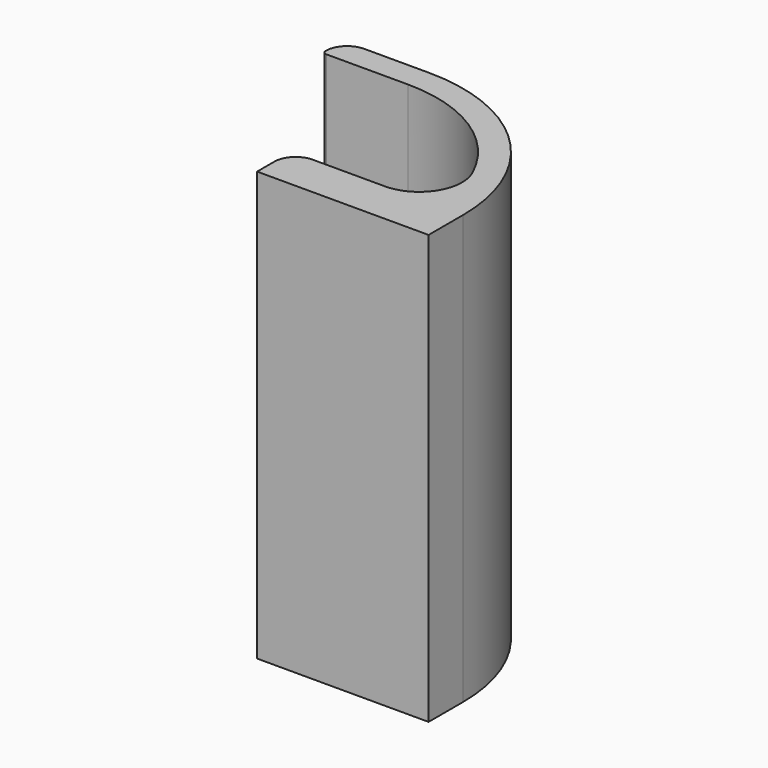
from build123d import *

# Parameters (mm, degrees)
F1_DEPTH = 50
F2_R     = 5
F3_R     = 2.5
F4_R     = 0.49999


# Not quite as in the source:
# - a fillet or chamfer is up to 0.001 mm smaller than in the source, because OpenCascade refuses the exact size


with BuildPart() as f1:
    # F0 (on Top) → F1 (new body)
    with BuildSketch(Plane.XY):
        with BuildLine():
            Line((7, 2.5), (10, 2.5))
            ThreePointArc((10, 2.5), (4.1421356237, 16.6421356237), (-10, 22.5))
            Line((-10, 22.5), (-20, 22.5))
            Line((-20, 22.5), (-20, 19.5))
            Line((-20, 19.5), (-10, 19.5))
            ThreePointArc((-10, 19.5), (2.0208152802, 14.5208152802), (7, 2.5))
        make_face()
        Polygon((-10, -2.5), (10, -2.5), (10, 2.5), (7, 2.5), (-10, 2.5), align=None)
    extrude(amount=F1_DEPTH)

    # F2
    f2_edges = [f1.edges().sort_by_distance(p)[0] for p in [
        (7, 2.5, 25),
    ]]
    fillet(f2_edges, radius=F2_R)

    # F3
    f3_edges = [f1.edges().sort_by_distance(p)[0] for p in [
        (-20, 22.5, 25),
        (-10, 2.5, 25),
    ]]
    fillet(f3_edges, radius=F3_R)

    # F4 (radius 0.5 in the source; OpenCascade refuses exactly that, so slightly less here)
    f4_edges = [f1.edges().sort_by_distance(p)[0] for p in [
        (-20, 19.5, 25),
    ]]
    fillet(f4_edges, radius=F4_R)


solid = f1.part
